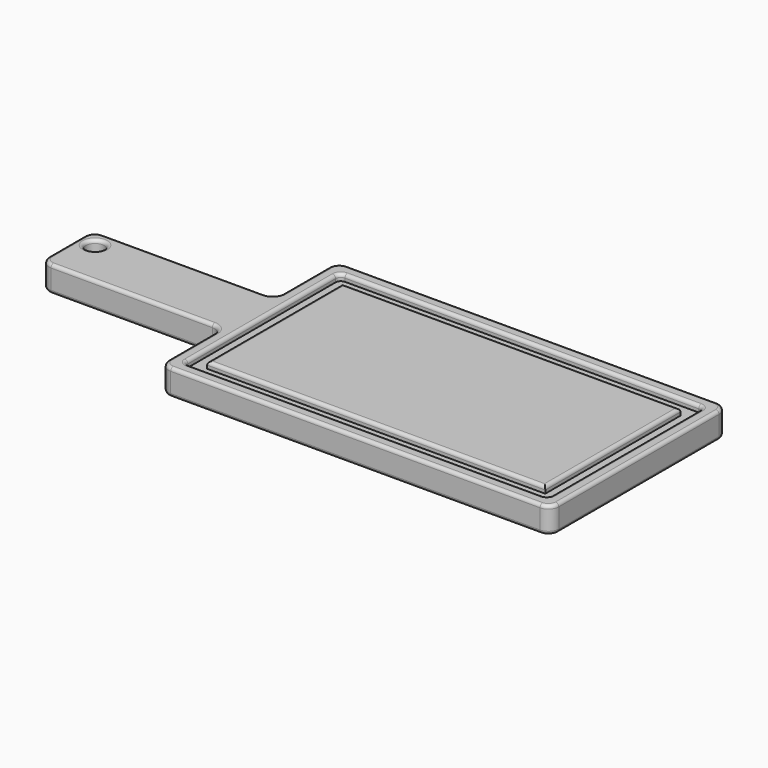
from build123d import *

# Parameters (mm, degrees)
F0_W         = 177.8
F0_H         = 63.5
F1_DEPTH     = 25.4
F2_R         = 8.89
F3_DEPTH     = 25.4
F5_DEPTH     = 6.35
F6_R         = 5.08
F7_R         = 10.16
F8_R         = 3.175
F9_TEXT_SIZE = 24.9454280398
F10_DEPTH    = 0.508


# Not quite as in the source:
# - Text() gives the source's letters only with a copy of the font that has no kerning and outlines rounded to 1/6400 em; it was checked with that copy


with BuildPart() as f1:
    # F0 (on Top) → F1 (new body)
    with BuildSketch(Plane.XY):
        Polygon((0, 76.2), (0, 0), (381, 0), (381, 215.9), (0, 215.9), (0, 139.7), align=None)
        with Locations((-88.9, 107.95)):
            Rectangle(F0_W, F0_H)
    extrude(amount=F1_DEPTH)

    # F2 (on face) → F3 (cut)
    with BuildSketch(Plane.XY.offset(25.4)):
        with Locations((-161.2977683544, 121.92)):
            Circle(F2_R)
    extrude(amount=-F3_DEPTH, mode=Mode.SUBTRACT)

    # F4 (on face) → F5 (cut)
    with BuildSketch(Plane.XY.offset(25.4)):
        Polygon((368.3, 203.2), (12.7, 203.2), (12.7, 127), (12.7, 101.6), (12.7, 12.7), (368.3, 12.7), align=None)
        Polygon((25.4, 101.6), (25.4, 127), (25.4, 190.5), (355.6, 190.5), (355.6, 25.4), (25.4, 25.4), align=None, mode=Mode.SUBTRACT)
    extrude(amount=-F5_DEPTH, mode=Mode.SUBTRACT)

    # F6
    f6_edges = [f1.edges().sort_by_distance(p)[0] for p in [
        (12.7, 203.2, 22.225),
        (12.7, 12.7, 22.225),
        (368.3, 12.7, 22.225),
        (368.3, 203.2, 22.225),
    ]]
    fillet(f6_edges, radius=F6_R)

    # F7
    f7_edges = [f1.edges().sort_by_distance(p)[0] for p in [
        (0, 215.9, 12.7),
        (0, 0, 12.7),
        (381, 0, 12.7),
        (381, 215.9, 12.7),
        (0, 139.7, 12.7),
        (0, 76.2, 12.7),
        (-177.8, 76.2, 12.7),
        (-177.8, 139.7, 12.7),
    ]]
    fillet(f7_edges, radius=F7_R)

    # F8
    f8_edges = [f1.edges().sort_by_distance(p)[0] for p in [
        (190.5, 190.5, 25.4),
        (355.6, 107.95, 25.4),
        (190.5, 25.4, 25.4),
        (25.4, 107.95, 25.4),
        (0, 38.1, 25.4),
        (-2.975795, 73.224205, 25.4),
        (2.975795, 2.975795, 25.4),
        (-88.9, 76.2, 25.4),
        (190.5, 0, 25.4),
        (-174.824205, 79.175795, 25.4),
        (378.024205, 2.975795, 25.4),
        (-177.8, 107.95, 25.4),
        (381, 107.95, 25.4),
        (-174.824205, 136.724205, 25.4),
        (378.024205, 212.924205, 25.4),
        (-88.9, 139.7, 25.4),
        (190.5, 215.9, 25.4),
        (-2.975795, 142.675795, 25.4),
        (2.975795, 212.924205, 25.4),
        (0, 177.8, 25.4),
        (190.5, 203.2, 25.4),
        (366.812102, 201.712102, 25.4),
        (14.187898, 201.712102, 25.4),
        (368.3, 107.95, 25.4),
        (12.7, 107.95, 25.4),
        (366.812102, 14.187898, 25.4),
        (14.187898, 14.187898, 25.4),
        (190.5, 12.7, 25.4),
        (-170.187768, 121.92, 25.4),
        (0, 38.1, 0),
        (-2.975795, 73.224205, 0),
        (2.975795, 2.975795, 0),
        (-88.9, 76.2, 0),
        (190.5, 0, 0),
        (-174.824205, 79.175795, 0),
        (378.024205, 2.975795, 0),
        (-177.8, 107.95, 0),
        (381, 107.95, 0),
        (-174.824205, 136.724205, 0),
        (378.024205, 212.924205, 0),
        (-88.9, 139.7, 0),
        (190.5, 215.9, 0),
        (-2.975795, 142.675795, 0),
        (2.975795, 212.924205, 0),
        (0, 177.8, 0),
        (-170.187768, 121.92, 0),
    ]]
    fillet(f8_edges, radius=F8_R)

    # F9 (on face) → F10 (join)
    with BuildSketch(Plane(origin=(0, 0, 0), x_dir=(1, 0, 0), z_dir=(0, 0, -1))):
        with Locations((30.7822384681, -44.6028790805)):
            Text('Jayden Masukawa', F9_TEXT_SIZE, font='Open Sans', font_style=FontStyle.ITALIC, text_align=(TextAlign.LEFT, TextAlign.BOTTOM))
    extrude(amount=F10_DEPTH)


solid = f1.part
